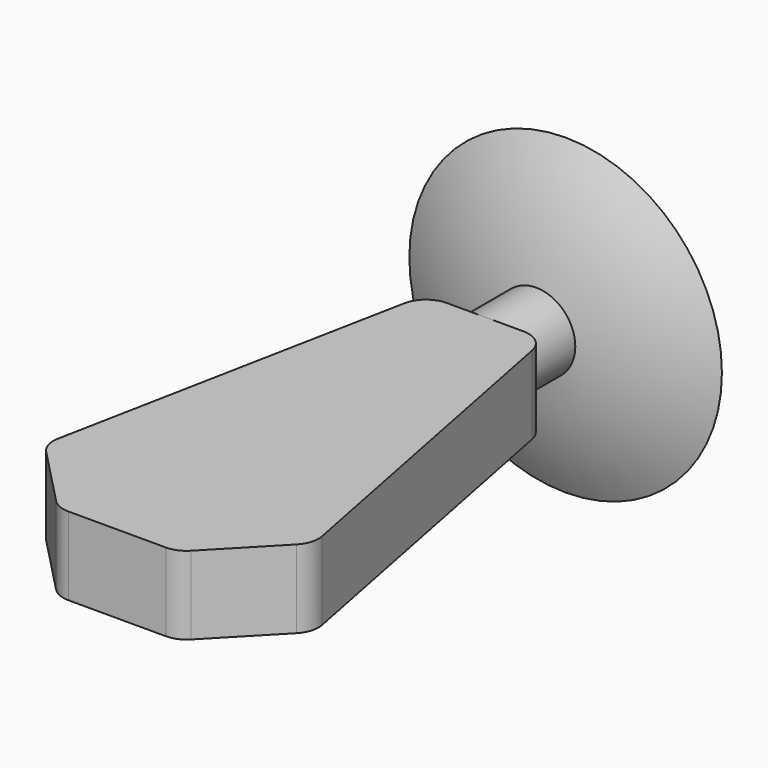
from build123d import *

# Parameters (mm, degrees)
F2_R     = 1.5
F3_DEPTH = 4
F5_DEPTH = 1.5


with BuildPart() as f1:
    # F0 (on Right) → F1 (revolve)
    with BuildSketch(Plane.YZ):
        with BuildLine():
            Line((0, 0), (0, 6))
            ThreePointArc((0, 6), (-1.1189941578, 3.0922762594), (-1.4995632221, 0))
            Line((-1.4995632221, 0), (0, 0))
        make_face()
    revolve(axis=Axis((0, 0.9339665994, 0), (0, 1, 0)))

    # F2 (on Front) → F3 (join)
    with BuildSketch(Plane.XZ):
        Circle(F2_R)
    extrude(amount=F3_DEPTH)

    # F4 (on Top) → F5 (join, symmetric)
    with BuildSketch(Plane.XY):
        with BuildLine():
            Line((1.4699705266, -3.8650664501), (0, -3.8650664501))
            Line((0, -3.8650664501), (-1.4699705266, -3.8650664501))
            ThreePointArc((-1.4699705266, -3.8650664501), (-2.105403361, -4.0929103047), (-2.4512772628, -4.6726162242))
            Line((-2.4512772628, -4.6726162242), (-5.0702010152, -18.0265497334))
            ThreePointArc((-5.0702010152, -18.0265497334), (-5.0479765813, -18.5021273815), (-4.8083588564, -18.913529096))
            Line((-4.8083588564, -18.913529096), (-2.5877873591, -21.213825008))
            ThreePointArc((-2.5877873591, -21.213825008), (-2.2591365885, -21.4397656254), (-1.8683227817, -21.5192958713))
            Line((-1.8683227817, -21.5192958713), (0, -21.5192958713))
            Line((0, -21.5192958713), (1.8683227817, -21.5192958713))
            ThreePointArc((1.8683227817, -21.5192958713), (2.2591365885, -21.4397656254), (2.5877873591, -21.213825008))
            Line((2.5877873591, -21.213825008), (4.8083588564, -18.913529096))
            ThreePointArc((4.8083588564, -18.913529096), (5.0479765813, -18.5021273815), (5.0702010152, -18.0265497334))
            Line((5.0702010152, -18.0265497334), (2.4512772628, -4.6726162242))
            ThreePointArc((2.4512772628, -4.6726162242), (2.105403361, -4.0929103047), (1.4699705266, -3.8650664501))
        make_face()
    extrude(amount=F5_DEPTH, both=True)


solid = f1.part
